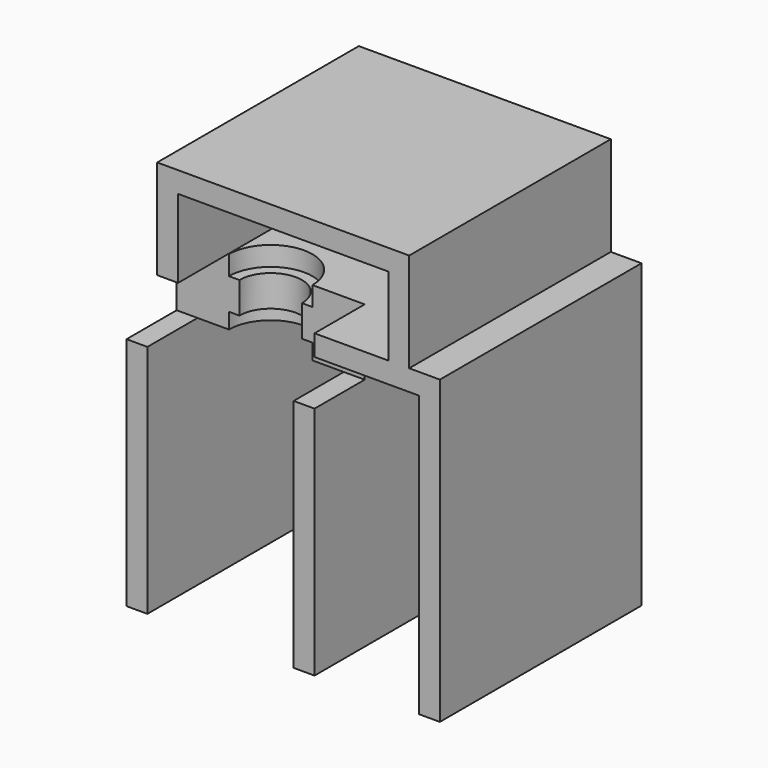
from build123d import *

# Parameters (mm, degrees)
F1_W     = 4
F1_H     = 15
F1_W_2   = 6
F1_H_2   = 6
F1_H_3   = 45
F2_DEPTH = 36.25
F4_DEPTH = 12


# Not quite as in the source:
# - a feature names something its author has since deleted; it is built from what else it names


with BuildPart() as f2:
    # F1 (on Front) → F2 (new body)
    with BuildSketch(Plane.XZ):
        Polygon((24.125, -2), (24.125, 2), (-24.125, 2), (-24.125, -2), (-20.125, -2), (20.125, -2), align=None)
        with Locations((-22.125, -9.5)):
            Rectangle(F1_W, F1_H)
        with Locations((22.125, -9.5)):
            Rectangle(F1_W, F1_H)
        Polygon((24.125, -21), (24.125, -17), (20.125, -17), (6, -17), (6, -21), align=None)
        Polygon((6, -21), (6, -17), (-4, -17), (-4, -20.7), (-6, -20.7), (-6, -26.7), (-4, -26.7), (-4, -29.7), (-0.85, -29.7), (2, -29.7), (6, -29.7), align=None)
        Polygon((-20.125, -17), (-24.125, -17), (-30, -17), (-30, -29.7), (-26, -29.7), (-23.15, -29.7), (-20, -29.7), (-20, -26.7), (-18, -26.7), (-18, -20.7), (-20, -20.7), (-20, -17), align=None)
        Polygon((-4, -20.7), (-4, -17), (-12, -17), (-12, -20.7), (-6, -20.7), align=None)
        Polygon((-12, -17), (-20, -17), (-20, -20.7), (-18, -20.7), (-12, -20.7), align=None)
        with Locations((-15, -23.7)):
            Rectangle(F1_W_2, F1_H_2)
        with Locations((-9, -23.7)):
            Rectangle(F1_W_2, F1_H_2)
        Polygon((-12, -29.7), (-12, -26.7), (-18, -26.7), (-20, -26.7), (-20, -29.7), align=None)
        Polygon((-6, -26.7), (-12, -26.7), (-12, -29.7), (-4, -29.7), (-4, -26.7), align=None)
        Polygon((30, -17), (24.125, -17), (24.125, -21), (26, -21), (26, -74.7), (30, -74.7), align=None)
        with Locations((-28, -52.2)):
            Rectangle(F1_W, F1_H_3)
        with Locations((4, -52.2)):
            Rectangle(F1_W, F1_H_3)
    extrude(amount=-F2_DEPTH)

    # F1 (on Front) → F3 (revolve, cut)
    with BuildSketch(Plane.XZ):
        Polygon((-12, -17), (-20, -17), (-20, -20.7), (-18, -20.7), (-12, -20.7), align=None)
        with Locations((-15, -23.7)):
            Rectangle(F1_W_2, F1_H_2)
        Polygon((-12, -29.7), (-12, -26.7), (-18, -26.7), (-20, -26.7), (-20, -29.7), align=None)
    revolve(axis=Axis((-12, 0, -48.15), (0, 0, -1)), mode=Mode.SUBTRACT)

    # F1 (on Front) → F4 (join)
    with BuildSketch(Plane.XZ):
        Polygon((24.125, -2), (24.125, 2), (-24.125, 2), (-24.125, -2), (-20.125, -2), (20.125, -2), align=None)
        with Locations((22.125, -9.5)):
            Rectangle(F1_W, F1_H)
        with Locations((-22.125, -9.5)):
            Rectangle(F1_W, F1_H)
        Polygon((24.125, -21), (24.125, -17), (20.125, -17), (6, -17), (6, -21), align=None)
        Polygon((30, -17), (24.125, -17), (24.125, -21), (26, -21), (26, -74.7), (30, -74.7), align=None)
        with Locations((-28, -52.2)):
            Rectangle(F1_W, F1_H_3)
        with Locations((4, -52.2)):
            Rectangle(F1_W, F1_H_3)
    extrude(amount=F4_DEPTH)


solid = f2.part
